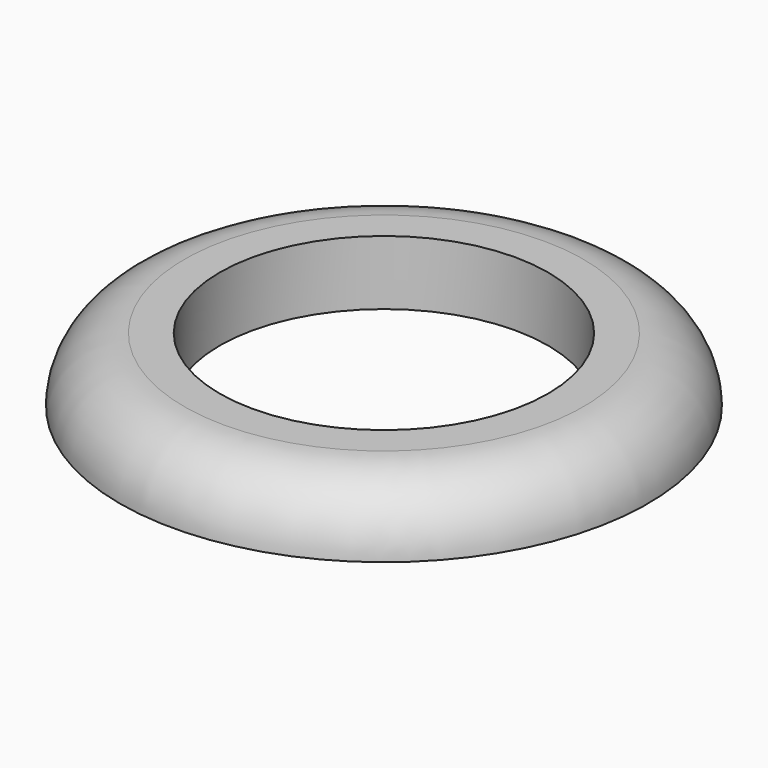
from build123d import *

# Parameters (mm, degrees)
F3_COPIES_COUNT = 4


# Not quite as in the source:
# - a pattern or mirror of a feature is missing from the dataset's text; its kind, count and spacing are read off the source's solid


with BuildPart() as f1:
    # F0 (on Right) → F1 (revolve)
    with BuildSketch(Plane.YZ):
        with BuildLine():
            Line((5.1, 2), (5.1, 0))
            Line((5.1, 0), (8.2, 0))
            ThreePointArc((8.2, 0), (7.6142135624, 1.4142135624), (6.2, 2))
            Line((6.2, 2), (5.1, 2))
        make_face()
    revolve(axis=Axis((0, 0, 1), (0, 0, 1)))

    # F2 (on Right) → F3 (revolve, cut)
    with BuildSketch(Plane.YZ):
        Polygon((-6.45, 0.5), (-6.7, 0.5), (-6.7, 0), (-5.7, 0), (-6.2, 1), align=None)
    f3 = revolve(axis=Axis((0, -6.7, 0.25), (0, 0, 1)), mode=Mode.SUBTRACT)

    # F3_copies: F3 ×4 about axis
    f3_copies_axis = Axis((0, 0, 0), (0, 0, 1))
    for i in range(1, F3_COPIES_COUNT):
        add(f3.rotate(f3_copies_axis, i * 360 / F3_COPIES_COUNT), mode=Mode.SUBTRACT)


solid = f1.part
